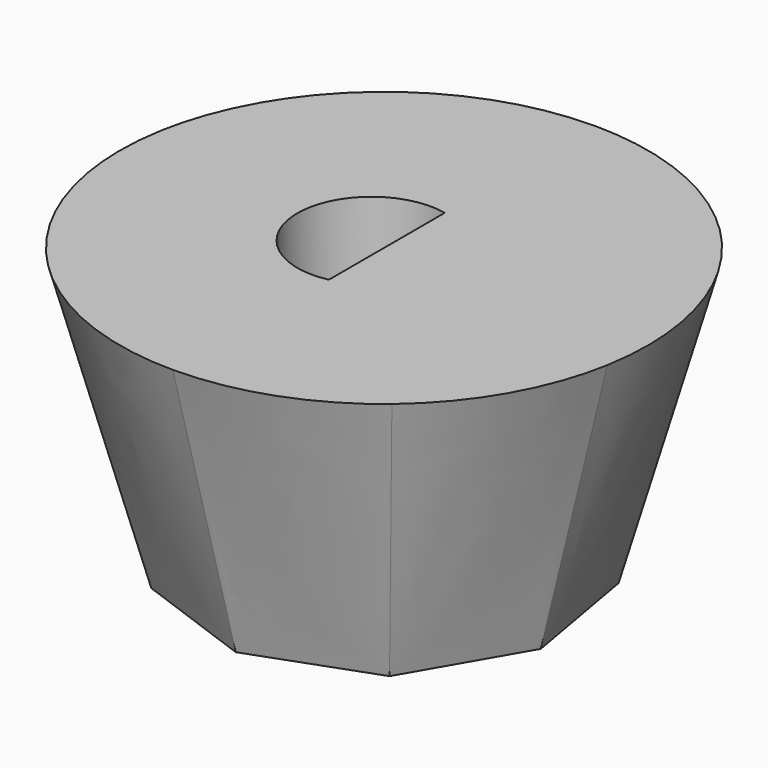
from build123d import *

# Parameters (mm, degrees)
F5_DEPTH = 10.414


# Not quite as in the source:
# - the arcs of a loft's sections are written as splines that run evenly, so that the points pair up as in the source's solid


with BuildPart() as f3:
    # F0 (on Top) → F3 section 0
    with BuildSketch(Plane.XY):
        Polygon((10.7835912141, -12.8513835704), (16.5214202528, -2.9131721502), (14.5286931401, 8.3881448954), (5.7378290387, 15.7645557206), (-5.7378290387, 15.7645557206), (-14.5286931401, 8.3881448954), (-16.5214202528, -2.9131721502), (-10.7835912141, -12.8513835704), (0, -16.7762897909), align=None)
    # F2 (on offset) → F3 section 1
    with BuildSketch(Plane.XY.offset(25.4)):
        with BuildLine():
            add(Edge.make_bspline(
                [(15.363307355, -18.3092767345), (17.4936884395, -16.5216747522), (19.3084205069, -14.3589612913), (22.0894355037, -9.5421020203), (23.0550342683, -6.8891412184), (23.5379524545, -4.1503760884)],
                knots=[0, 0, 0, 0, 0.5, 0.5, 1, 1, 1, 1], degree=3))
            add(Edge.make_bspline(
                [(23.5379524545, -4.1503760884), (24.0208706408, -1.4116109583), (24.0208706408, 1.4116109583), (23.0550342683, 6.8891412184), (22.0894355037, 9.5421020203), (20.6989280053, 11.9505316558)],
                knots=[0, 0, 0, 0, 0.5, 0.5, 1, 1, 1, 1], degree=3))
            add(Edge.make_bspline(
                [(20.6989280053, 11.9505316558), (19.3084205069, 14.3589612913), (17.4936884395, 16.5216747522), (13.2329262705, 20.0968787168), (10.7879443702, 21.5084896751), (8.1746450995, 22.4596528229)],
                knots=[0, 0, 0, 0, 0.5, 0.5, 1, 1, 1, 1], degree=3))
            add(Edge.make_bspline(
                [(8.1746450995, 22.4596528229), (5.5613458287, 23.4108159707), (2.7810149968, 23.9010633116), (-2.7810149968, 23.9010633116), (-5.5613458287, 23.4108159707), (-8.1746450995, 22.4596528229)],
                knots=[0, 0, 0, 0, 0.5, 0.5, 1, 1, 1, 1], degree=3))
            add(Edge.make_bspline(
                [(-8.1746450995, 22.4596528229), (-10.7879443702, 21.5084896751), (-13.2329262705, 20.0968787168), (-17.4936884395, 16.5216747522), (-19.3084205069, 14.3589612913), (-20.6989280053, 11.9505316558)],
                knots=[0, 0, 0, 0, 0.5, 0.5, 1, 1, 1, 1], degree=3))
            add(Edge.make_bspline(
                [(-20.6989280053, 11.9505316558), (-22.0894355037, 9.5421020203), (-23.0550342683, 6.8891412184), (-24.0208706408, 1.4116109583), (-24.0208706408, -1.4116109583), (-23.5379524545, -4.1503760884)],
                knots=[0, 0, 0, 0, 0.5, 0.5, 1, 1, 1, 1], degree=3))
            add(Edge.make_bspline(
                [(-23.5379524545, -4.1503760884), (-23.0550342683, -6.8891412184), (-22.0894355037, -9.5421020203), (-19.3084205069, -14.3589612913), (-17.4936884395, -16.5216747522), (-15.363307355, -18.3092767345)],
                knots=[0, 0, 0, 0, 0.5, 0.5, 1, 1, 1, 1], degree=3))
            add(Edge.make_bspline(
                [(-15.363307355, -18.3092767345), (-13.2329262705, -20.0968787168), (-10.7879443702, -21.5084896751), (-5.5613458287, -23.4108159707), (-2.7810149968, -23.9010633116), (0, -23.9010633116)],
                knots=[0, 0, 0, 0, 0.5, 0.5, 1, 1, 1, 1], degree=3))
            add(Edge.make_bspline(
                [(0, -23.9010633116), (2.7810149968, -23.9010633116), (5.5613458287, -23.4108159707), (10.7879443702, -21.5084896751), (13.2329262705, -20.0968787168), (15.363307355, -18.3092767345)],
                knots=[0, 0, 0, 0, 0.5, 0.5, 1, 1, 1, 1], degree=3))
        make_face()
    loft(ruled=True)

    # F4 (on face) → F5 (cut)
    with BuildSketch(Plane.XY.offset(25.4)):
        with BuildLine():
            Line((0, -6.2373387627), (0, 6.8825809285))
            ThreePointArc((0, 6.8825809285), (-8.1053000761, 0.3226210829), (0, -6.2373387627))
        make_face()
    extrude(amount=-F5_DEPTH, mode=Mode.SUBTRACT)


solid = f3.part
